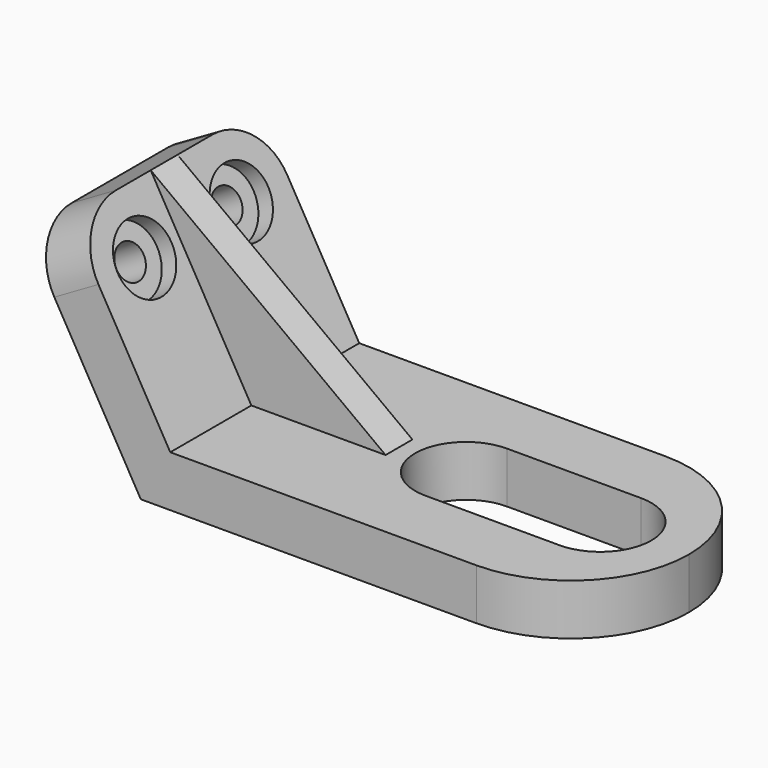
from build123d import *

# Parameters (mm, degrees)
F1_DEPTH  = 44.704
F3_R      = 22.35199
F5_R      = 10.922
F4_R      = 3.175
F6_DEPTH  = 28.5637839421
F4_R_2    = 6.35
F7_DEPTH  = 3.175
F8_DEPTH  = 9.653
F11_DEPTH = 3.175


# Not quite as in the source:
# - a fillet or chamfer is up to 0.001 mm smaller than in the source, because OpenCascade refuses the exact size


with BuildPart() as f1:
    # F0 (on Front) → F1 (new body)
    with BuildSketch(Plane.XZ):
        Polygon((-21.8362923991, 37.8215678842), (0, 0), (85.852, 0), (85.852, 9.652), (30.9725847982, 9.652), (5.5725847982, 9.652), (-13.4774152018, 42.6475678842), align=None)
    extrude(amount=F1_DEPTH)

    # F3 (radius 22.352 in the source; OpenCascade refuses exactly that, so slightly less here)
    f3_edges = [f1.edges().sort_by_distance(p)[0] for p in [
        (85.852, -44.704, 4.826),
        (85.852, 0, 4.826),
    ]]
    fillet(f3_edges, radius=F3_R)

    # F5
    f5_edges = [f1.edges().sort_by_distance(p)[0] for p in [
        (-17.656854, -44.704, 40.234568),
        (-17.656854, 0, 40.234568),
    ]]
    fillet(f5_edges, radius=F5_R)

    # F4 (on face) → F6 (cut, through all)
    with BuildSketch(Plane(origin=(8.3588771973, 0, 4.826), x_dir=(0, 1, 0), z_dir=(0.8660254038, 0, 0.5))):
        with Locations((-33.782, 32.7505847982)):
            Circle(F4_R)
        with Locations((-10.922, 32.7505847982)):
            Circle(F4_R)
    extrude(amount=-F6_DEPTH, mode=Mode.SUBTRACT)

    # F4 (on face) → F7 (cut)
    with BuildSketch(Plane(origin=(8.3588771973, 0, 4.826), x_dir=(0, 1, 0), z_dir=(0.8660254038, 0, 0.5))):
        with Locations((-33.782, 32.7505847982)):
            Circle(F4_R_2)
        with Locations((-33.782, 32.7505847982)):
            Circle(F4_R, mode=Mode.SUBTRACT)
        with Locations((-10.922, 32.7505847982)):
            Circle(F4_R_2)
        with Locations((-10.922, 32.7505847982)):
            Circle(F4_R, mode=Mode.SUBTRACT)
    extrude(amount=-F7_DEPTH, mode=Mode.SUBTRACT)

    # F2 (on face) → F8 (cut, through all)
    with BuildSketch(Plane.XY.offset(9.652)):
        with BuildLine():
            Line((43.6725847982, -32.004), (69.0725847982, -32.004))
            ThreePointArc((69.0725847982, -32.004), (78.7245847982, -22.352), (69.0725847982, -12.7))
            Line((69.0725847982, -12.7), (43.6725847982, -12.7))
            ThreePointArc((43.6725847982, -12.7), (34.0205847982, -22.352), (43.6725847982, -32.004))
        make_face()
    extrude(amount=-F8_DEPTH, mode=Mode.SUBTRACT)

    # F10 (on offset) → F11 (join, symmetric)
    with BuildSketch(Plane.XZ.offset(22.352)):
        Polygon((30.9725847982, 9.652), (-13.4774152018, 42.6475678842), (-8.0164152018, 33.1888384241), (5.5725847982, 9.652), align=None)
    extrude(amount=F11_DEPTH, both=True)


solid = f1.part
